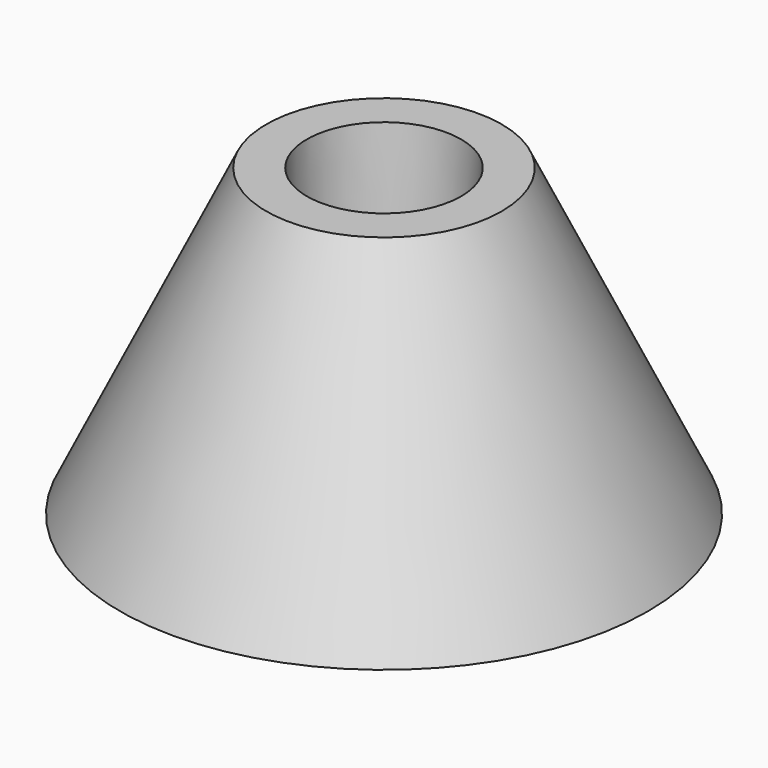
from build123d import *


# Not quite as in the source:
# - a fillet or chamfer that OpenCascade refuses, or shapes differently, is made with other operations: its cross-section is extruded or revolved along the edge and cut away or added


with BuildPart() as f1:
    # F0 (on Front) → F1 (revolve)
    with BuildSketch(Plane.XZ):
        Polygon((64.667229809, 0), (65, 0), (29, 75), (19, 75), (17.3, 44), (16.3, 44), (0, 15.7675718366), (0, 15.1675718366), (16.3, 43.4), (17.8679982822, 43.4), (19.5679982822, 74.4), (28.955229809, 74.4), align=None)
    revolve(axis=Axis((0, 0, 43.4963169246), (0, 0, -1)))

    # F2: fillet of radius 1.5 on 1 edges, made by hand

    # F2_s1 → F2_t2 (revolve)
    with BuildSketch(Plane.XZ):
        with BuildLine():
            ThreePointArc((17.3744099359, 45.3568870669), (17.0526414639, 44.5078566678), (16.3, 44))
            Line((16.3, 44), (16.3084667935, 43.9712195655))
            ThreePointArc((16.3084667935, 43.9712195655), (16.8, 43.97), (17.3, 43.97))
            Line((17.3, 43.97), (17.3299549922, 43.9983573069))
            Line((17.3299549922, 43.9983573069), (17.4043649282, 45.3552443738))
            Line((17.4043649282, 45.3552443738), (17.3744099359, 45.3568870669))
        make_face()
    revolve(axis=Axis((0, 0, 44), (0, 0, -1)))


solid = f1.part
